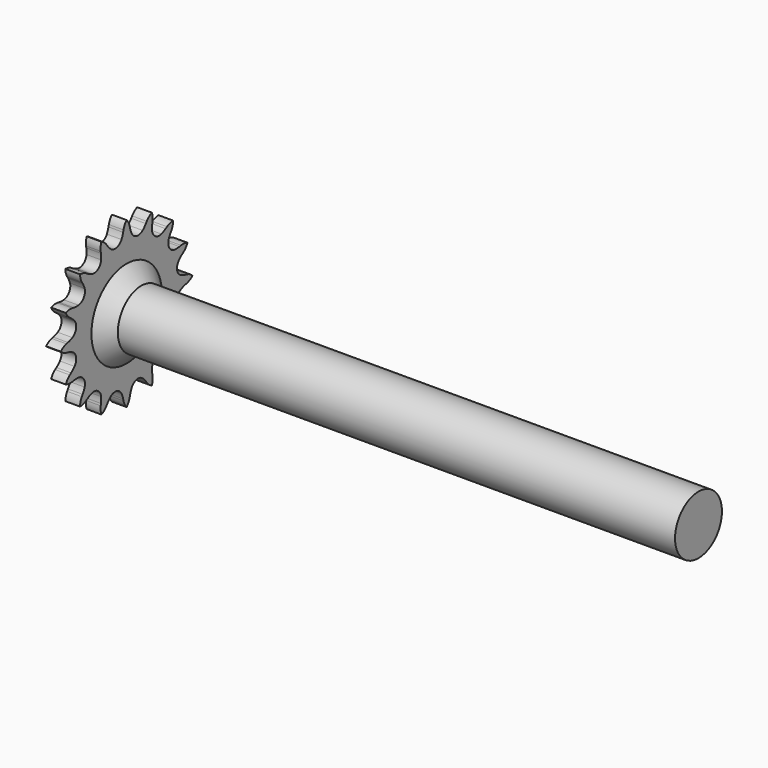
from build123d import *

# Parameters (mm, degrees)
F0_W     = 12.7
F0_H     = 12.7
F0_H_2   = 38.1
F2_R     = 25.4
F3_DEPTH = 508
F6_DEPTH = 508.001
F7_SIZE  = 12.69999


# Not quite as in the source:
# - a fillet or chamfer is up to 0.001 mm smaller than in the source, because OpenCascade refuses the exact size


with BuildPart() as f1:
    # F0 (on Front) → F1 (revolve)
    with BuildSketch(Plane.XZ):
        with Locations((6.35, 31.75)):
            Rectangle(F0_W, F0_H)
        with Locations((19.05, 31.75)):
            Rectangle(F0_W, F0_H)
        with Locations((6.35, 57.15)):
            Rectangle(F0_W, F0_H_2)
        with Locations((19.05, -31.75)):
            Rectangle(F0_W, F0_H)
        with Locations((6.35, -31.75)):
            Rectangle(F0_W, F0_H)
        with Locations((6.35, -57.15)):
            Rectangle(F0_W, F0_H_2)
    revolve(axis=Axis((27.5155087221, 0, 0), (1, 0, 0)))


with BuildPart() as f3:
    # F2 (on face) → F3 (new body)
    with BuildSketch(Plane(origin=(0, 0, 0), x_dir=(0, -1, 0), z_dir=(-1, 0, 0))):
        Circle(F2_R)
    extrude(amount=-F3_DEPTH)

    # F4: union F1
    add(f1.part)

    # F5 (on face) → F6 (intersect, through all)
    with BuildSketch(Plane(origin=(0, 0, 0), x_dir=(0, -1, 0), z_dir=(-1, 0, 0))):
        with BuildLine():
            ThreePointArc((5.5316382467, 58.7105467237), (4.4969254374, 61.0482621798), (3.7655024898, 63.497867173))
            Line((3.7655024898, 63.497867173), (3.381355787, 65.1617893485))
            ThreePointArc((3.381355787, 65.1617893485), (2.117661135, 68.4688843406), (0, 71.3060154229))
            ThreePointArc((0, 71.3060154229), (-2.117661135, 68.4688843406), (-3.381355787, 65.1617893485))
            Line((-3.381355787, 65.1617893485), (-3.7655024898, 63.497867173))
            ThreePointArc((-3.7655024898, 63.497867173), (-4.4969254374, 61.0482621798), (-5.5316382467, 58.7105467237))
            ThreePointArc((-5.5316382467, 58.7105467237), (-10.8801864977, 54.6983912614), (-17.3569861789, 56.3583387714))
            ThreePointArc((-17.3569861789, 56.3583387714), (-19.20754114, 58.1221387847), (-20.8207110777, 60.1053752566))
            Line((-20.8207110777, 60.1053752566), (-21.8123718032, 61.4956323195))
            ThreePointArc((-21.8123718032, 61.4956323195), (-24.2454438902, 64.0673946879), (-27.2876307303, 65.8781681941))
            ThreePointArc((-27.2876307303, 65.8781681941), (-28.1583714491, 62.4466070245), (-28.0603026107, 58.9076546423))
            Line((-28.0603026107, 58.9076546423), (-27.7784524376, 57.2233844219))
            ThreePointArc((-27.7784524376, 57.2233844219), (-27.5167758818, 54.6803410618), (-27.5781208937, 52.1246061497))
            ThreePointArc((-27.5781208937, 52.1246061497), (-30.9841497278, 46.371057034), (-37.6031668002, 45.4260846308))
            ThreePointArc((-37.6031668002, 45.4260846308), (-39.9878336957, 46.3474466383), (-42.2371601238, 47.562384814))
            Line((-42.2371601238, 47.562384814), (-43.685363516, 48.4673227291))
            ThreePointArc((-43.685363516, 48.4673227291), (-46.9173998687, 49.9122249664), (-50.4209670449, 50.4209670449))
            ThreePointArc((-50.4209670449, 50.4209670449), (-49.9122249664, 46.9173998687), (-48.4673227291, 43.685363516))
            Line((-48.4673227291, 43.685363516), (-47.562384814, 42.2371601238))
            ThreePointArc((-47.562384814, 42.2371601238), (-46.3474466383, 39.9878336957), (-45.4260846308, 37.6031668002))
            ThreePointArc((-45.4260846308, 37.6031668002), (-46.371057034, 30.9841497278), (-52.1246061497, 27.5781208937))
            ThreePointArc((-52.1246061497, 27.5781208937), (-54.6803410618, 27.5167758818), (-57.2233844219, 27.7784524376))
            Line((-57.2233844219, 27.7784524376), (-58.9076546423, 28.0603026107))
            ThreePointArc((-58.9076546423, 28.0603026107), (-62.4466070245, 28.1583714491), (-65.8781681941, 27.2876307303))
            ThreePointArc((-65.8781681941, 27.2876307303), (-64.0673946879, 24.2454438902), (-61.4956323195, 21.8123718032))
            Line((-61.4956323195, 21.8123718032), (-60.1053752566, 20.8207110777))
            ThreePointArc((-60.1053752566, 20.8207110777), (-58.1221387847, 19.20754114), (-56.3583387714, 17.3569861789))
            ThreePointArc((-56.3583387714, 17.3569861789), (-54.6983912614, 10.8801864977), (-58.7105467237, 5.5316382467))
            ThreePointArc((-58.7105467237, 5.5316382467), (-61.0482621798, 4.4969254374), (-63.497867173, 3.7655024898))
            Line((-63.497867173, 3.7655024898), (-65.1617893485, 3.381355787))
            ThreePointArc((-65.1617893485, 3.381355787), (-68.4688843406, 2.117661135), (-71.3060154229, 0))
            ThreePointArc((-71.3060154229, 0), (-68.4688843406, -2.117661135), (-65.1617893485, -3.381355787))
            Line((-65.1617893485, -3.381355787), (-63.497867173, -3.7655024898))
            ThreePointArc((-63.497867173, -3.7655024898), (-61.0482621798, -4.4969254374), (-58.7105467237, -5.5316382467))
            ThreePointArc((-58.7105467237, -5.5316382467), (-54.6983912614, -10.8801864977), (-56.3583387714, -17.3569861789))
            ThreePointArc((-56.3583387714, -17.3569861789), (-58.1221387847, -19.20754114), (-60.1053752566, -20.8207110777))
            Line((-60.1053752566, -20.8207110777), (-61.4956323195, -21.8123718032))
            ThreePointArc((-61.4956323195, -21.8123718032), (-64.0673946879, -24.2454438902), (-65.8781681941, -27.2876307303))
            ThreePointArc((-65.8781681941, -27.2876307303), (-62.4466070245, -28.1583714491), (-58.9076546423, -28.0603026107))
            Line((-58.9076546423, -28.0603026107), (-57.2233844219, -27.7784524376))
            ThreePointArc((-57.2233844219, -27.7784524376), (-54.6803410618, -27.5167758818), (-52.1246061497, -27.5781208937))
            ThreePointArc((-52.1246061497, -27.5781208937), (-46.371057034, -30.9841497278), (-45.4260846308, -37.6031668002))
            ThreePointArc((-45.4260846308, -37.6031668002), (-46.3474466383, -39.9878336957), (-47.562384814, -42.2371601238))
            Line((-47.562384814, -42.2371601238), (-48.4673227291, -43.685363516))
            ThreePointArc((-48.4673227291, -43.685363516), (-49.9122249664, -46.9173998687), (-50.4209670449, -50.4209670449))
            ThreePointArc((-50.4209670449, -50.4209670449), (-46.9173998687, -49.9122249664), (-43.685363516, -48.4673227291))
            Line((-43.685363516, -48.4673227291), (-42.2371601238, -47.562384814))
            ThreePointArc((-42.2371601238, -47.562384814), (-39.9878336957, -46.3474466383), (-37.6031668002, -45.4260846308))
            ThreePointArc((-37.6031668002, -45.4260846308), (-30.9841497278, -46.371057034), (-27.5781208937, -52.1246061497))
            ThreePointArc((-27.5781208937, -52.1246061497), (-27.5167758818, -54.6803410618), (-27.7784524376, -57.2233844219))
            Line((-27.7784524376, -57.2233844219), (-28.0603026107, -58.9076546423))
            ThreePointArc((-28.0603026107, -58.9076546423), (-28.1583714491, -62.4466070245), (-27.2876307303, -65.8781681941))
            ThreePointArc((-27.2876307303, -65.8781681941), (-24.2454438902, -64.0673946879), (-21.8123718032, -61.4956323195))
            Line((-21.8123718032, -61.4956323195), (-20.8207110777, -60.1053752566))
            ThreePointArc((-20.8207110777, -60.1053752566), (-19.20754114, -58.1221387847), (-17.3569861789, -56.3583387714))
            ThreePointArc((-17.3569861789, -56.3583387714), (-10.8801864977, -54.6983912614), (-5.5316382467, -58.7105467237))
            ThreePointArc((-5.5316382467, -58.7105467237), (-4.4969254374, -61.0482621798), (-3.7655024898, -63.497867173))
            Line((-3.7655024898, -63.497867173), (-3.381355787, -65.1617893485))
            ThreePointArc((-3.381355787, -65.1617893485), (-2.117661135, -68.4688843406), (0, -71.3060154229))
            ThreePointArc((0, -71.3060154229), (2.117661135, -68.4688843406), (3.381355787, -65.1617893485))
            Line((3.381355787, -65.1617893485), (3.7655024898, -63.497867173))
            ThreePointArc((3.7655024898, -63.497867173), (4.4969254374, -61.0482621798), (5.5316382467, -58.7105467237))
            ThreePointArc((5.5316382467, -58.7105467237), (10.8801864977, -54.6983912614), (17.3569861789, -56.3583387714))
            ThreePointArc((17.3569861789, -56.3583387714), (19.20754114, -58.1221387847), (20.8207110777, -60.1053752566))
            Line((20.8207110777, -60.1053752566), (21.8123718032, -61.4956323195))
            ThreePointArc((21.8123718032, -61.4956323195), (24.2454438902, -64.0673946879), (27.2876307303, -65.8781681941))
            ThreePointArc((27.2876307303, -65.8781681941), (28.1583714491, -62.4466070245), (28.0603026107, -58.9076546423))
            Line((28.0603026107, -58.9076546423), (27.7784524376, -57.2233844219))
            ThreePointArc((27.7784524376, -57.2233844219), (27.5167758818, -54.6803410618), (27.5781208937, -52.1246061497))
            ThreePointArc((27.5781208937, -52.1246061497), (30.9841497278, -46.371057034), (37.6031668002, -45.4260846308))
            ThreePointArc((37.6031668002, -45.4260846308), (39.9878336957, -46.3474466383), (42.2371601238, -47.562384814))
            Line((42.2371601238, -47.562384814), (43.685363516, -48.4673227291))
            ThreePointArc((43.685363516, -48.4673227291), (46.9173998687, -49.9122249664), (50.4209670449, -50.4209670449))
            ThreePointArc((50.4209670449, -50.4209670449), (49.9122249664, -46.9173998687), (48.4673227291, -43.685363516))
            Line((48.4673227291, -43.685363516), (47.562384814, -42.2371601238))
            ThreePointArc((47.562384814, -42.2371601238), (46.3474466383, -39.9878336957), (45.4260846308, -37.6031668002))
            ThreePointArc((45.4260846308, -37.6031668002), (46.371057034, -30.9841497278), (52.1246061497, -27.5781208937))
            ThreePointArc((52.1246061497, -27.5781208937), (54.6803410618, -27.5167758818), (57.2233844219, -27.7784524376))
            Line((57.2233844219, -27.7784524376), (58.9076546423, -28.0603026107))
            ThreePointArc((58.9076546423, -28.0603026107), (62.4466070245, -28.1583714491), (65.8781681941, -27.2876307303))
            ThreePointArc((65.8781681941, -27.2876307303), (64.0673946879, -24.2454438902), (61.4956323195, -21.8123718032))
            Line((61.4956323195, -21.8123718032), (60.1053752566, -20.8207110777))
            ThreePointArc((60.1053752566, -20.8207110777), (58.1221387847, -19.20754114), (56.3583387714, -17.3569861789))
            ThreePointArc((56.3583387714, -17.3569861789), (54.6983912614, -10.8801864977), (58.7105467237, -5.5316382467))
            ThreePointArc((58.7105467237, -5.5316382467), (61.0482621798, -4.4969254374), (63.497867173, -3.7655024898))
            Line((63.497867173, -3.7655024898), (65.1617893485, -3.381355787))
            ThreePointArc((65.1617893485, -3.381355787), (68.4688843406, -2.117661135), (71.3060154229, 0))
            ThreePointArc((71.3060154229, 0), (68.4688843406, 2.117661135), (65.1617893485, 3.381355787))
            Line((65.1617893485, 3.381355787), (63.497867173, 3.7655024898))
            ThreePointArc((63.497867173, 3.7655024898), (61.0482621798, 4.4969254374), (58.7105467237, 5.5316382467))
            ThreePointArc((58.7105467237, 5.5316382467), (54.6983912614, 10.8801864977), (56.3583387714, 17.3569861789))
            ThreePointArc((56.3583387714, 17.3569861789), (58.1221387847, 19.20754114), (60.1053752566, 20.8207110777))
            Line((60.1053752566, 20.8207110777), (61.4956323195, 21.8123718032))
            ThreePointArc((61.4956323195, 21.8123718032), (64.0673946879, 24.2454438902), (65.8781681941, 27.2876307303))
            ThreePointArc((65.8781681941, 27.2876307303), (62.4466070245, 28.1583714491), (58.9076546423, 28.0603026107))
            Line((58.9076546423, 28.0603026107), (57.2233844219, 27.7784524376))
            ThreePointArc((57.2233844219, 27.7784524376), (54.6803410618, 27.5167758818), (52.1246061497, 27.5781208937))
            ThreePointArc((52.1246061497, 27.5781208937), (46.371057034, 30.9841497278), (45.4260846308, 37.6031668002))
            ThreePointArc((45.4260846308, 37.6031668002), (46.3474466383, 39.9878336957), (47.562384814, 42.2371601238))
            Line((47.562384814, 42.2371601238), (48.4673227291, 43.685363516))
            ThreePointArc((48.4673227291, 43.685363516), (49.9122249664, 46.9173998687), (50.4209670449, 50.4209670449))
            ThreePointArc((50.4209670449, 50.4209670449), (46.9173998687, 49.9122249664), (43.685363516, 48.4673227291))
            Line((43.685363516, 48.4673227291), (42.2371601238, 47.562384814))
            ThreePointArc((42.2371601238, 47.562384814), (39.9878336957, 46.3474466383), (37.6031668002, 45.4260846308))
            ThreePointArc((37.6031668002, 45.4260846308), (30.9841497278, 46.371057034), (27.5781208937, 52.1246061497))
            ThreePointArc((27.5781208937, 52.1246061497), (27.5167758818, 54.6803410618), (27.7784524376, 57.2233844219))
            Line((27.7784524376, 57.2233844219), (28.0603026107, 58.9076546423))
            ThreePointArc((28.0603026107, 58.9076546423), (28.1583714491, 62.4466070245), (27.2876307303, 65.8781681941))
            ThreePointArc((27.2876307303, 65.8781681941), (24.2454438902, 64.0673946879), (21.8123718032, 61.4956323195))
            Line((21.8123718032, 61.4956323195), (20.8207110777, 60.1053752566))
            ThreePointArc((20.8207110777, 60.1053752566), (19.20754114, 58.1221387847), (17.3569861789, 56.3583387714))
            ThreePointArc((17.3569861789, 56.3583387714), (10.8801864977, 54.6983912614), (5.5316382467, 58.7105467237))
        make_face()
    extrude(amount=-F6_DEPTH, mode=Mode.INTERSECT)

    # F7 (size 12.7 in the source; OpenCascade refuses exactly that, so slightly less here)
    f7_edges = [f3.edges().sort_by_distance(p)[0] for p in [
        (25.4, 0, -38.1),
    ]]
    chamfer(f7_edges, length=F7_SIZE)


solid = f3.part
